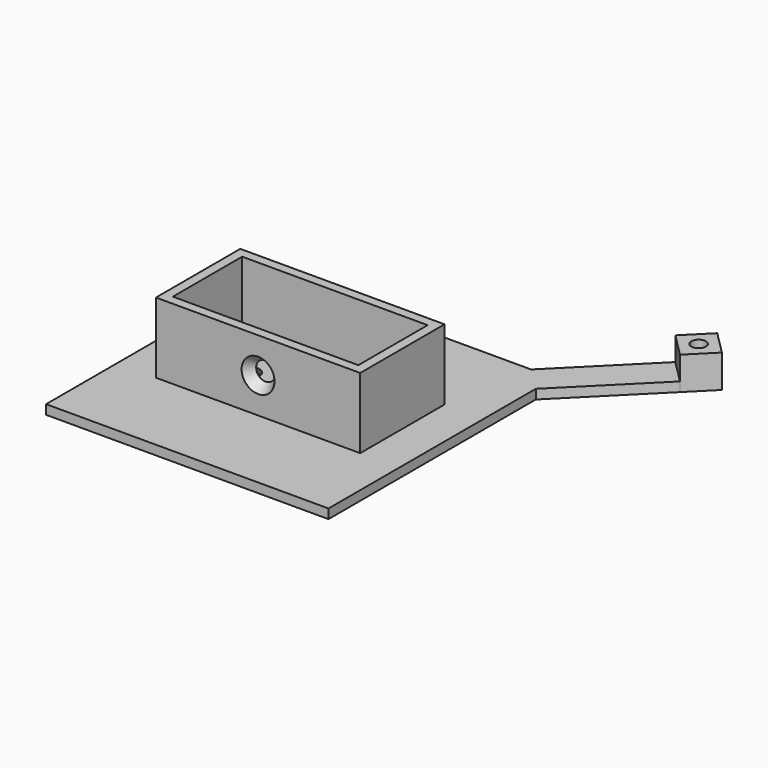
from build123d import *

# Parameters (mm, degrees)
F0_W      = 60
F0_H      = 60
F0_W_2    = 43.4
F0_H_2    = 22.4
F0_W_3    = 39.4
F0_H_3    = 18.4
F0_R      = 2
F1_DEPTH  = 2
F2_R      = 1.55
F3_DEPTH  = 2
F4_DEPTH  = 15
F5_R      = 3.5
F7_R      = 3.5
F8_R      = 2
F10_DEPTH = 5


# Not quite as in the source:
# - a pattern or mirror of a feature is missing from the dataset's text; its kind, count and spacing are read off the source's solid
# - a feature names something its author has since deleted; it is built from what else it names


with BuildPart() as f1:
    # F0 (on Top) → F1 (new body)
    with BuildSketch(Plane.XY):
        Rectangle(F0_W, F0_H)
        Rectangle(F0_W_2, F0_H_2, mode=Mode.SUBTRACT)
        Rectangle(F0_W_2, F0_H_2)
        Rectangle(F0_W_3, F0_H_3, mode=Mode.SUBTRACT)
        Rectangle(F0_W_3, F0_H_3)
        with Locations((-10.6629617512, 0)):
            Circle(F0_R, mode=Mode.SUBTRACT)
        with Locations((-10.6629617512, 0)):
            Circle(F0_R)
    extrude(amount=-F1_DEPTH)

    # F2 (on Top) → F3 (join)
    with BuildSketch(Plane.XY):
        Polygon((42.0728534806, 47.0226009489), (-2.4748737342, 2.4748737342), (2.4748737342, -2.4748737342), (47.0226009489, 42.0728534806), align=None)
        Polygon((47.0226009489, 51.9723484172), (42.0728534806, 47.0226009489), (47.0226009489, 42.0728534806), (51.9723484172, 47.0226009489), align=None)
        with Locations((47.0226009489, 47.0226009489)):
            Circle(F2_R, mode=Mode.SUBTRACT)
        with Locations((47.0226009489, 47.0226009489)):
            Circle(F2_R)
    extrude(amount=-F3_DEPTH)

    # F0 (on Top) → F4 (join)
    with BuildSketch(Plane.XY):
        Rectangle(F0_W_2, F0_H_2)
        Rectangle(F0_W_3, F0_H_3, mode=Mode.SUBTRACT)
    extrude(amount=F4_DEPTH)

    # F0 (on Top) → F6 section 0
    with BuildSketch(Plane.XY):
        with Locations((-10.6629617512, 0)):
            Circle(F0_R)
    # F5 (on face) → F6 section 1
    with BuildSketch(Plane(origin=(0, 0, -2), x_dir=(1, 0, 0), z_dir=(0, 0, -1))):
        with Locations((-10.6629617512, 0)):
            Circle(F5_R)
    f6 = loft(mode=Mode.SUBTRACT)

    # F6_copies: F6 across plane
    add(f6.mirror(Plane(origin=(0, 0, 0), x_dir=(0, 0, 1), z_dir=(1, 0, 0))), mode=Mode.SUBTRACT)

    # F7 (on face) → F9 section 0
    with BuildSketch(Plane.XZ.offset(11.2)):
        with Locations((0, 7.5)):
            Circle(F7_R)
    # F8 (on face) → F9 section 1
    with BuildSketch(Plane(origin=(0, -9.2, 0), x_dir=(-1, 0, 0), z_dir=(0, 1, 0))):
        with Locations((0, 7.5)):
            Circle(F8_R)
    loft(mode=Mode.SUBTRACT)

    # F2 (on Top) → F10 (join)
    with BuildSketch(Plane.XY):
        Polygon((47.0226009489, 51.9723484172), (42.0728534806, 47.0226009489), (47.0226009489, 42.0728534806), (51.9723484172, 47.0226009489), align=None)
        with Locations((47.0226009489, 47.0226009489)):
            Circle(F2_R, mode=Mode.SUBTRACT)
    extrude(amount=F10_DEPTH)


solid = f1.part
